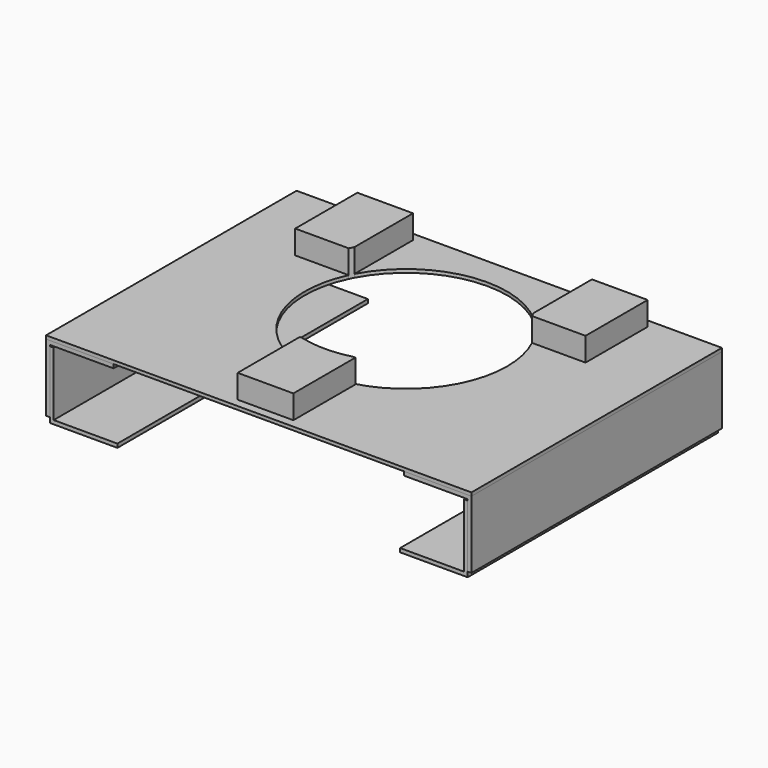
from build123d import *

# Parameters (mm, degrees)
F0_W          = 252
F0_H          = 185.5
F1_DEPTH      = 2
F3_DEPTH      = 157.5
F3_DEPTH_BACK = 28
F8_DEPTH      = 16
F9_D          = 9


with BuildPart() as f1:
    # F0 (on Top) → F1 (new body)
    with BuildSketch(Plane.XY):
        with Locations((0, 64.75)):
            Rectangle(F0_W, F0_H)
        with BuildLine():
            ThreePointArc((-53, 135.3309518948), (-52.2518116893, 132.4580398915), (-52, 129.5))
            ThreePointArc((-52, 129.5), (-52.2518116893, 126.5419601085), (-53, 123.6690481052))
            Line((-53, 123.6690481052), (-53, 109.1247222208))
            ThreePointArc((-53, 109.1247222208), (0, 141), (53, 109.1247222209))
            Line((53, 109.1247222209), (53, 123.6690481052))
            ThreePointArc((53, 123.6690481052), (52, 129.5), (53, 135.3309518948))
            Line((53, 135.3309518948), (53, 152.5))
            Line((53, 152.5), (86, 152.5))
            Line((86, 152.5), (86, 135.3309518948))
            ThreePointArc((86, 135.3309518948), (86.7481883107, 132.4580398915), (87, 129.5))
            ThreePointArc((87, 129.5), (86.7481883107, 126.5419601085), (86, 123.6690481052))
            Line((86, 123.6690481052), (86, 106.5))
            Line((86, 106.5), (54.3116009707, 106.5))
            ThreePointArc((54.3116009707, 106.5), (58.5606354911, 94.0633828268), (60, 81))
            ThreePointArc((60, 81), (47.548593511, 44.4058576391), (15.3622914957, 23))
            Line((15.3622914957, 23), (16.5, 23))
            Line((16.5, 23), (16.5, 5.8309518948))
            ThreePointArc((16.5, 5.8309518948), (17.2481883107, 2.9580398915), (17.5, 0))
            ThreePointArc((17.5, 0), (17.2481883107, -2.9580398915), (16.5, -5.8309518948))
            Line((16.5, -5.8309518948), (16.5, -23))
            Line((16.5, -23), (-16.5, -23))
            Line((-16.5, -23), (-16.5, -5.8309518948))
            ThreePointArc((-16.5, -5.8309518948), (-17.5, 0), (-16.5, 5.8309518948))
            Line((-16.5, 5.8309518948), (-16.5, 23))
            Line((-16.5, 23), (-15.3622914957, 23))
            ThreePointArc((-15.3622914957, 23), (-54.3753190598, 55.6361541334), (-54.3116009707, 106.5))
            Line((-54.3116009707, 106.5), (-86, 106.5))
            Line((-86, 106.5), (-86, 123.6690481052))
            ThreePointArc((-86, 123.6690481052), (-87, 129.5), (-86, 135.3309518948))
            Line((-86, 135.3309518948), (-86, 152.5))
            Line((-86, 152.5), (-53, 152.5))
            Line((-53, 152.5), (-53, 135.3309518948))
        make_face(mode=Mode.SUBTRACT)
        with BuildLine():
            Line((-53, 123.6690481052), (-53, 135.3309518948))
            ThreePointArc((-53, 135.3309518948), (-69.5, 147), (-86, 135.3309518948))
            Line((-86, 135.3309518948), (-86, 123.6690481052))
            ThreePointArc((-86, 123.6690481052), (-69.5, 112), (-53, 123.6690481052))
        make_face()
        with BuildLine():
            Line((53, 135.3309518948), (53, 123.6690481052))
            ThreePointArc((53, 123.6690481052), (69.5, 112), (86, 123.6690481052))
            Line((86, 123.6690481052), (86, 135.3309518948))
            ThreePointArc((86, 135.3309518948), (69.5, 147), (53, 135.3309518948))
        make_face()
        with BuildLine():
            ThreePointArc((16.5, 5.8309518948), (0, 17.5), (-16.5, 5.8309518948))
            Line((-16.5, 5.8309518948), (-16.5, -5.8309518948))
            ThreePointArc((-16.5, -5.8309518948), (0, -17.5), (16.5, -5.8309518948))
            Line((16.5, -5.8309518948), (16.5, 5.8309518948))
        make_face()
        with BuildLine():
            ThreePointArc((-86, 135.3309518948), (-69.5, 147), (-53, 135.3309518948))
            Line((-53, 135.3309518948), (-53, 152.5))
            Line((-53, 152.5), (-86, 152.5))
            Line((-86, 152.5), (-86, 135.3309518948))
        make_face()
        with BuildLine():
            Line((53, 152.5), (53, 135.3309518948))
            ThreePointArc((53, 135.3309518948), (69.5, 147), (86, 135.3309518948))
            Line((86, 135.3309518948), (86, 152.5))
            Line((86, 152.5), (53, 152.5))
        make_face()
        with BuildLine():
            ThreePointArc((16.5, -5.8309518948), (0, -17.5), (-16.5, -5.8309518948))
            Line((-16.5, -5.8309518948), (-16.5, -23))
            Line((-16.5, -23), (16.5, -23))
            Line((16.5, -23), (16.5, -5.8309518948))
        make_face()
        with BuildLine():
            Line((-53, 109.1247222208), (-53, 123.6690481052))
            ThreePointArc((-53, 123.6690481052), (-69.5, 112), (-86, 123.6690481052))
            Line((-86, 123.6690481052), (-86, 106.5))
            Line((-86, 106.5), (-54.3116009707, 106.5))
            ThreePointArc((-54.3116009707, 106.5), (-53.6718475312, 107.820379986), (-53, 109.1247222208))
        make_face()
        with BuildLine():
            Line((53, 123.6690481052), (53, 109.1247222209))
            ThreePointArc((53, 109.1247222209), (53.6718475312, 107.820379986), (54.3116009707, 106.5))
            Line((54.3116009707, 106.5), (86, 106.5))
            Line((86, 106.5), (86, 123.6690481052))
            ThreePointArc((86, 123.6690481052), (69.5, 112), (53, 123.6690481052))
        make_face()
        with BuildLine():
            ThreePointArc((15.3622914957, 23), (0, 21), (-15.3622914957, 23))
            Line((-15.3622914957, 23), (-16.5, 23))
            Line((-16.5, 23), (-16.5, 5.8309518948))
            ThreePointArc((-16.5, 5.8309518948), (0, 17.5), (16.5, 5.8309518948))
            Line((16.5, 5.8309518948), (16.5, 23))
            Line((16.5, 23), (15.3622914957, 23))
        make_face()
        with BuildLine():
            ThreePointArc((-53, 123.6690481052), (-52.2518116893, 126.5419601085), (-52, 129.5))
            ThreePointArc((-52, 129.5), (-52.2518116893, 132.4580398915), (-53, 135.3309518948))
            Line((-53, 135.3309518948), (-53, 123.6690481052))
        make_face()
        with BuildLine():
            Line((-86, 123.6690481052), (-86, 135.3309518948))
            ThreePointArc((-86, 135.3309518948), (-87, 129.5), (-86, 123.6690481052))
        make_face()
        with BuildLine():
            ThreePointArc((53, 135.3309518948), (52, 129.5), (53, 123.6690481052))
            Line((53, 123.6690481052), (53, 135.3309518948))
        make_face()
        with BuildLine():
            Line((86, 135.3309518948), (86, 123.6690481052))
            ThreePointArc((86, 123.6690481052), (86.7481883107, 126.5419601085), (87, 129.5))
            ThreePointArc((87, 129.5), (86.7481883107, 132.4580398915), (86, 135.3309518948))
        make_face()
        with BuildLine():
            Line((-16.5, -5.8309518948), (-16.5, 5.8309518948))
            ThreePointArc((-16.5, 5.8309518948), (-17.5, 0), (-16.5, -5.8309518948))
        make_face()
        with BuildLine():
            ThreePointArc((17.5, 0), (17.2481883107, 2.9580398915), (16.5, 5.8309518948))
            Line((16.5, 5.8309518948), (16.5, -5.8309518948))
            ThreePointArc((16.5, -5.8309518948), (17.2481883107, -2.9580398915), (17.5, 0))
        make_face()
    extrude(amount=F1_DEPTH)

    # F9 (through all)
    with Locations(Plane(origin=(0, 0, 0), x_dir=(1, 0, 0), z_dir=(0, 0, -1))):
        with Locations((-69.5, -129.5), (69.5, -129.5), (0, 0)):
            Hole(F9_D / 2)


with BuildPart() as f3:
    # F2 (on Front) → F3 (new body, two sides)
    with BuildSketch(Plane.XZ) as f3_sk:
        Polygon((-86, 0), (-126, 0), (-126, -40), (-123.75, -40), (-123.75, -2.25), (-86, -2.25), align=None)
    extrude(amount=-F3_DEPTH)
    extrude(f3_sk.sketch, amount=F3_DEPTH_BACK)


with BuildPart() as f3b:
    # F2 (on Front) → F3, piece 2 (new body, two sides)
    with BuildSketch(Plane.XZ) as f3_2_sk:
        Polygon((126, 0), (86, 0), (86, -2.25), (123.75, -2.25), (123.75, -40), (126, -40), align=None)
    extrude(amount=-F3_DEPTH)
    extrude(f3_2_sk.sketch, amount=F3_DEPTH_BACK)


with BuildPart() as f4_1:
    # F4: instance of F3
    add(f3.part.mirror(Plane(origin=(124.875, 64.75, -40), x_dir=(1, 0, 0), z_dir=(0, 0, -1))))


with BuildPart() as f4_2:
    # F4: instance of F3b
    add(f3b.part.mirror(Plane(origin=(124.875, 64.75, -40), x_dir=(1, 0, 0), z_dir=(0, 0, -1))))


with BuildPart() as f4_1_1:
    # F5: moved
    add(f4_1.part.moved(Location((2.25, 0, 37))))


with BuildPart() as f7_1:
    # F7: instance of F4_1
    add(f4_1_1.part.mirror(Plane.YZ))


with BuildPart() as f8:
    # F0 (on Top) → F8 (new body)
    with BuildSketch(Plane.XY):
        with BuildLine():
            Line((-53, 123.6690481052), (-53, 135.3309518948))
            ThreePointArc((-53, 135.3309518948), (-69.5, 147), (-86, 135.3309518948))
            Line((-86, 135.3309518948), (-86, 123.6690481052))
            ThreePointArc((-86, 123.6690481052), (-69.5, 112), (-53, 123.6690481052))
        make_face()
        with BuildLine():
            ThreePointArc((-86, 135.3309518948), (-69.5, 147), (-53, 135.3309518948))
            Line((-53, 135.3309518948), (-53, 152.5))
            Line((-53, 152.5), (-86, 152.5))
            Line((-86, 152.5), (-86, 135.3309518948))
        make_face()
        with BuildLine():
            Line((-53, 109.1247222208), (-53, 123.6690481052))
            ThreePointArc((-53, 123.6690481052), (-69.5, 112), (-86, 123.6690481052))
            Line((-86, 123.6690481052), (-86, 106.5))
            Line((-86, 106.5), (-54.3116009707, 106.5))
            ThreePointArc((-54.3116009707, 106.5), (-53.6718475312, 107.820379986), (-53, 109.1247222208))
        make_face()
    extrude(amount=F8_DEPTH)


with BuildPart() as f8b:
    # F0 (on Top) → F8, piece 2 (new body)
    with BuildSketch(Plane.XY):
        with BuildLine():
            Line((53, 123.6690481052), (53, 109.1247222209))
            ThreePointArc((53, 109.1247222209), (53.6718475312, 107.820379986), (54.3116009707, 106.5))
            Line((54.3116009707, 106.5), (86, 106.5))
            Line((86, 106.5), (86, 123.6690481052))
            ThreePointArc((86, 123.6690481052), (69.5, 112), (53, 123.6690481052))
        make_face()
        with BuildLine():
            Line((53, 135.3309518948), (53, 123.6690481052))
            ThreePointArc((53, 123.6690481052), (69.5, 112), (86, 123.6690481052))
            Line((86, 123.6690481052), (86, 135.3309518948))
            ThreePointArc((86, 135.3309518948), (69.5, 147), (53, 135.3309518948))
        make_face()
        with BuildLine():
            Line((53, 152.5), (53, 135.3309518948))
            ThreePointArc((53, 135.3309518948), (69.5, 147), (86, 135.3309518948))
            Line((86, 135.3309518948), (86, 152.5))
            Line((86, 152.5), (53, 152.5))
        make_face()
    extrude(amount=F8_DEPTH)


with BuildPart() as f8c:
    # F0 (on Top) → F8, piece 3 (new body)
    with BuildSketch(Plane.XY):
        with BuildLine():
            ThreePointArc((15.3622914957, 23), (0, 21), (-15.3622914957, 23))
            Line((-15.3622914957, 23), (-16.5, 23))
            Line((-16.5, 23), (-16.5, 5.8309518948))
            ThreePointArc((-16.5, 5.8309518948), (0, 17.5), (16.5, 5.8309518948))
            Line((16.5, 5.8309518948), (16.5, 23))
            Line((16.5, 23), (15.3622914957, 23))
        make_face()
        with BuildLine():
            ThreePointArc((16.5, 5.8309518948), (0, 17.5), (-16.5, 5.8309518948))
            Line((-16.5, 5.8309518948), (-16.5, -5.8309518948))
            ThreePointArc((-16.5, -5.8309518948), (0, -17.5), (16.5, -5.8309518948))
            Line((16.5, -5.8309518948), (16.5, 5.8309518948))
        make_face()
        with BuildLine():
            ThreePointArc((16.5, -5.8309518948), (0, -17.5), (-16.5, -5.8309518948))
            Line((-16.5, -5.8309518948), (-16.5, -23))
            Line((-16.5, -23), (16.5, -23))
            Line((16.5, -23), (16.5, -5.8309518948))
        make_face()
    extrude(amount=F8_DEPTH)


solid = Compound([f1.part, f3.part, f3b.part, f4_1_1.part, f7_1.part, f8.part, f8b.part, f8c.part])
